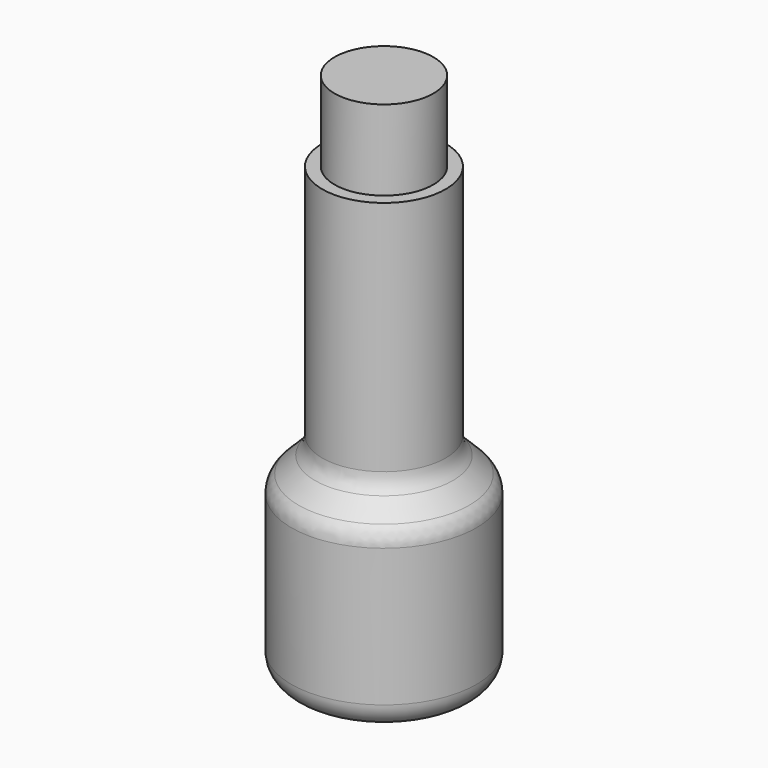
from build123d import *

# Parameters (mm, degrees)
F2_R         = 2
F3_TEXT_SIZE = 10.4166666667
F4_DEPTH     = 2


# Not quite as in the source:
# - Text() gives the source's letters only with a copy of the font that has no kerning and outlines rounded to 1/6400 em; it was checked with that copy


with BuildPart() as f1:
    # F0 (on Right) → F1 (revolve)
    with BuildSketch(Plane.YZ):
        Polygon((-7.5, 0), (0, 0), (0, 43), (-4, 43), (-4, 36.5), (-5, 36.5), (-5, 16.5), (-7.5, 14), align=None)
    revolve(axis=Axis((0, 0, 21.5), (0, 0, -1)))

    # F2
    f2_edges = [f1.edges().sort_by_distance(p)[0] for p in [
        (0, 7.5, 0),
        (0, 7.5, 14),
        (0, 5, 16.5),
    ]]
    fillet(f2_edges, radius=F2_R)

    # F3 (on face) → F4 (cut)
    with BuildSketch(Plane(origin=(0, 0, 0), x_dir=(1, 0, 0), z_dir=(0, 0, -1))):
        with Locations((-3.3526070786, -3.4768432774)):
            Text('B', F3_TEXT_SIZE, font='Arimo', font_style=FontStyle.BOLD, text_align=(TextAlign.LEFT, TextAlign.BOTTOM))
    extrude(amount=-F4_DEPTH, mode=Mode.SUBTRACT)


solid = f1.part
